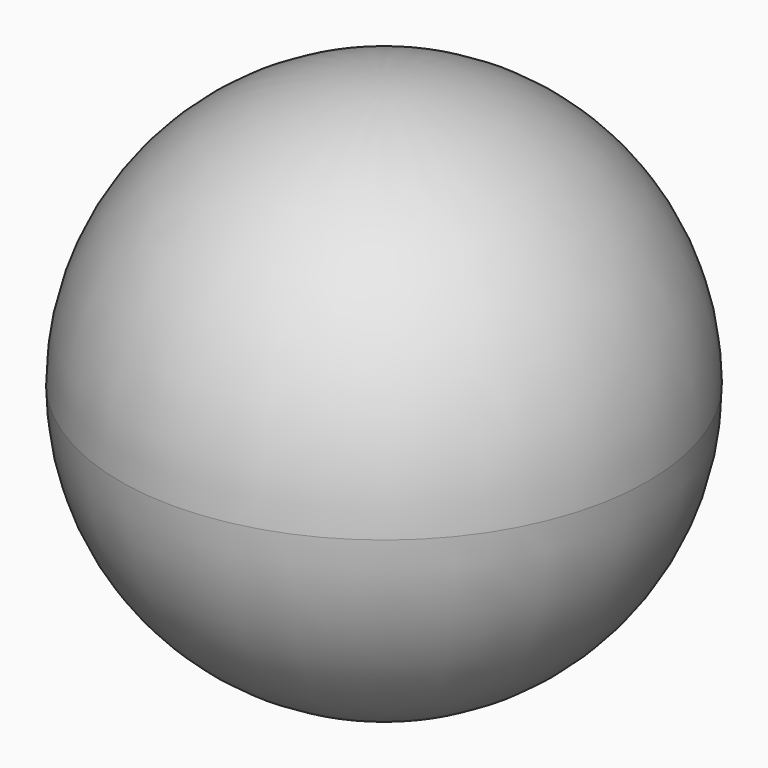
from build123d import *

# Parameters (mm, degrees)
F0_R     = 63.5
F1_DEPTH = 127
F2_R     = 63.49999


# Not quite as in the source:
# - a fillet or chamfer is up to 0.001 mm smaller than in the source, because OpenCascade refuses the exact size


with BuildPart() as f1:
    # F0 (on Top) → F1 (new body)
    with BuildSketch(Plane.XY):
        Circle(F0_R)
    extrude(amount=F1_DEPTH)

    # F2 (radius 63.5 in the source; OpenCascade refuses exactly that, so slightly less here)
    f2_edges = [f1.edges().sort_by_distance(p)[0] for p in [
        (-63.5, 0, 127),
        (63.5, 0, 63.5),
        (-63.5, 0, 0),
    ]]
    fillet(f2_edges, radius=F2_R)


solid = f1.part
